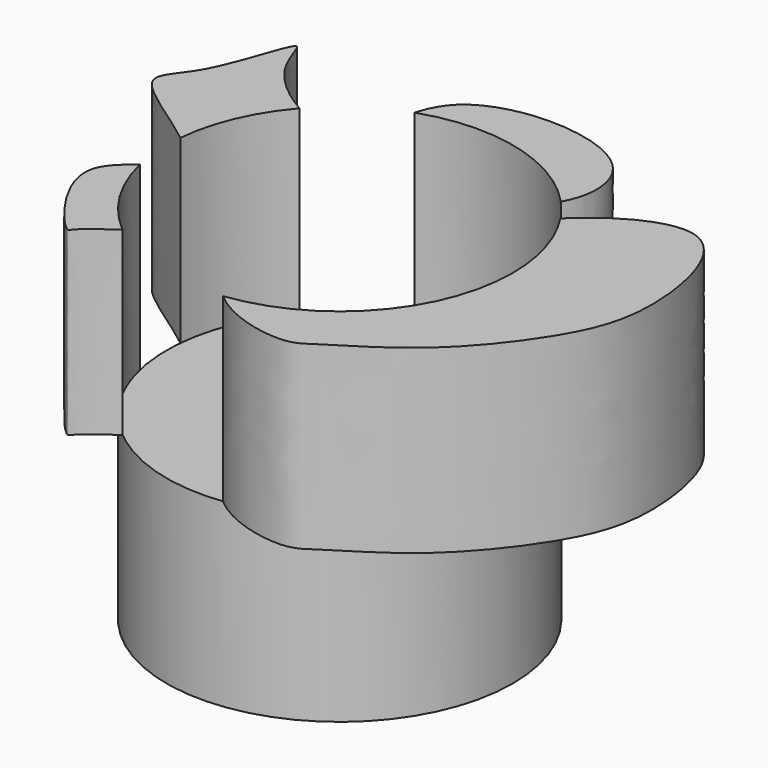
from build123d import *

# Parameters (mm, degrees)
F0_R     = 23.9546443397
F1_DEPTH = 25
F3_DEPTH = 25


with BuildPart() as f1:
    # F0 (on Top) → F1 (new body)
    with BuildSketch(Plane.XY):
        Circle(F0_R)
    extrude(amount=F1_DEPTH)


with BuildPart() as f3:
    # F2 (on face) → F3 (new body)
    with BuildSketch(Plane.XY.offset(25)):
        with BuildLine():
            add(Edge.make_bspline(
                [(-24.7150976211, 21.3320404291), (-23.2002903756, 19.186358509), (-20.6654275959, 17.0985687847), (-18.0975842985, 15.6940252326)],
                knots=[0, 0, 0, 0, 0.0212956958, 0.0212956958, 0.0212956958, 0.0212956958], degree=3))
            add(Edge.make_bspline(
                [(-23.8481216764, 2.2565633053), (-27.4560942193, 5.1533829377), (-37.6616802367, 10.9856760089), (-30.9990816465, 14.9718419563), (-27.2416588005, 31.1404224602), (-26.7158251233, 24.1660147459), (-24.7150976211, 21.3320404291)],
                knots=[0.8728036995, 0.8728036995, 0.8728036995, 0.8728036995, 0.9051808039, 0.9331614819, 0.9718730655, 1, 1, 1, 1], degree=3))
            ThreePointArc((-23.8481216764, 2.2565633053), (-22.0227588688, 9.4245995803), (-18.0975842985, 15.6940252326))
        make_face()
    extrude(amount=F3_DEPTH)


with BuildPart() as f3b:
    # F2 (on face) → F3, piece 2 (new body)
    with BuildSketch(Plane.XY.offset(25)):
        with BuildLine():
            add(Edge.make_bspline(
                [(-7.798120177, 22.6498191416), (-7.3357771288, 24.1640022303), (-3.8961489999, 31.7139758191), (19.1628892215, 31.0167173164), (19.4173730169, 19.4670823497), (17.5636049801, 16.2894065437)],
                knots=[0.0736423478, 0.0736423478, 0.0736423478, 0.0736423478, 0.0864536893, 0.1399292421, 0.1703739198, 0.1703739198, 0.1703739198, 0.1703739198], degree=3))
            ThreePointArc((-7.798120177, 22.6498191416), (5.8270820712, 23.2351049057), (17.5636049801, 16.2894065437))
        make_face()
    extrude(amount=F3_DEPTH)


with BuildPart() as f3c:
    # F2 (on face) → F3, piece 3 (new body)
    with BuildSketch(Plane.XY.offset(25)):
        with BuildLine():
            ThreePointArc((-15.2805750437, -18.4480083418), (-20.3976980009, -12.5602110535), (-23.3517529855, -5.3404698245))
            add(Edge.make_bspline(
                [(-15.2805750437, -18.4480083418), (-17.2835096748, -19.7258473209), (-19.7184054128, -21.7136067449), (-19.8127175625, -23.0306574397), (-30.2600566586, -10.9709624007), (-24.8443676836, -6.5218797636), (-23.3517529855, -5.3404698245)],
                knots=[0.7503882685, 0.7503882685, 0.7503882685, 0.7503882685, 0.7685108982, 0.7778578374, 0.8205387441, 0.8384697352, 0.8384697352, 0.8384697352, 0.8384697352], degree=3))
        make_face()
    extrude(amount=F3_DEPTH)


with BuildPart() as f3d:
    # F2 (on face) → F3, piece 4 (new body)
    with BuildSketch(Plane.XY.offset(25)):
        with BuildLine():
            add(Edge.make_bspline(
                [(19.9944816312, 13.1926377098), (24.3380571596, 17.4099341736), (36.9154241585, 24.2242234648), (41.826872761, 2.8912504159), (37.7503183518, -8.245948549), (27.9109539258, -20.4495389333), (18.0849304531, -25.7934387672), (14.8437220967, -28.7013705154), (6.3842665907, -26.8969779377), (2.8987011595, -23.7786146996)],
                knots=[0.4163295284, 0.4163295284, 0.4163295284, 0.4163295284, 0.4537574098, 0.499996756, 0.5404228804, 0.5850869705, 0.622204964, 0.6447753293, 0.6846222223, 0.6846222223, 0.6846222223, 0.6846222223], degree=3))
            ThreePointArc((19.9944816312, 13.1926377098), (22.9432526212, 6.887099869), (23.9546443397, 0))
            ThreePointArc((23.9546443397, 0), (17.9340784648, -15.8806112937), (2.8987011595, -23.7786146996))
        make_face()
    extrude(amount=F3_DEPTH)


solid = Compound([f1.part, f3.part, f3b.part, f3c.part, f3d.part])
